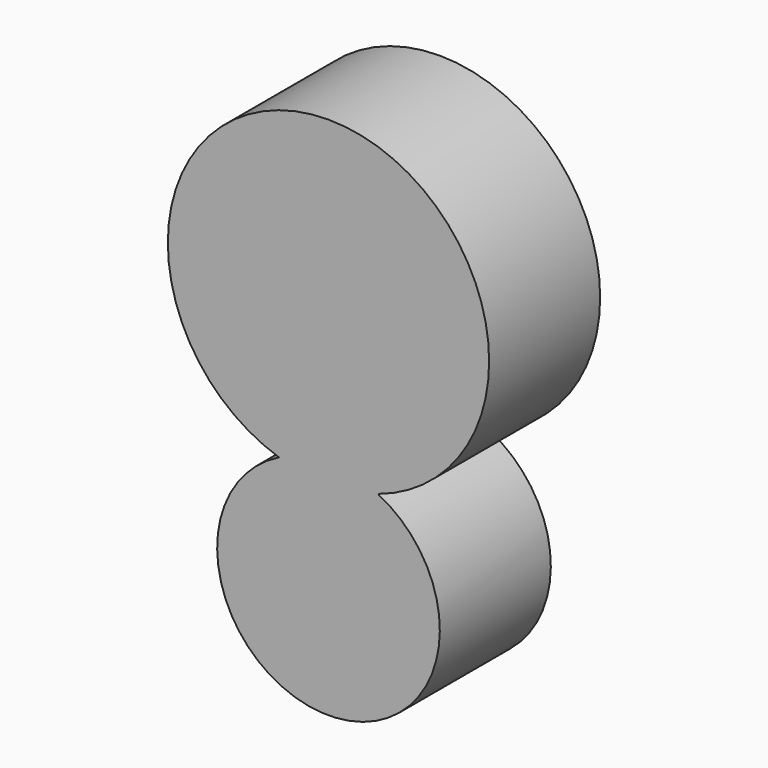
from build123d import *

# Parameters (mm, degrees)
F0_R     = 20.3761943404
F1_DEPTH = 25.4
F2_R     = 29.4019202889
F3_DEPTH = 25.4


# Not quite as in the source:
# - the program builds the solid bodies; features that only make, move or delete a surface that nothing else refers to are left out


with BuildPart() as f1:
    # F0 (on Front) → F1 (new body)
    with BuildSketch(Plane.XZ):
        Circle(F0_R)
    extrude(amount=F1_DEPTH)

    # F2 (on Front) → F3 (join)
    with BuildSketch(Plane.XZ):
        with Locations((0, 46.2284311652)):
            Circle(F2_R)
    extrude(amount=F3_DEPTH)


solid = f1.part
